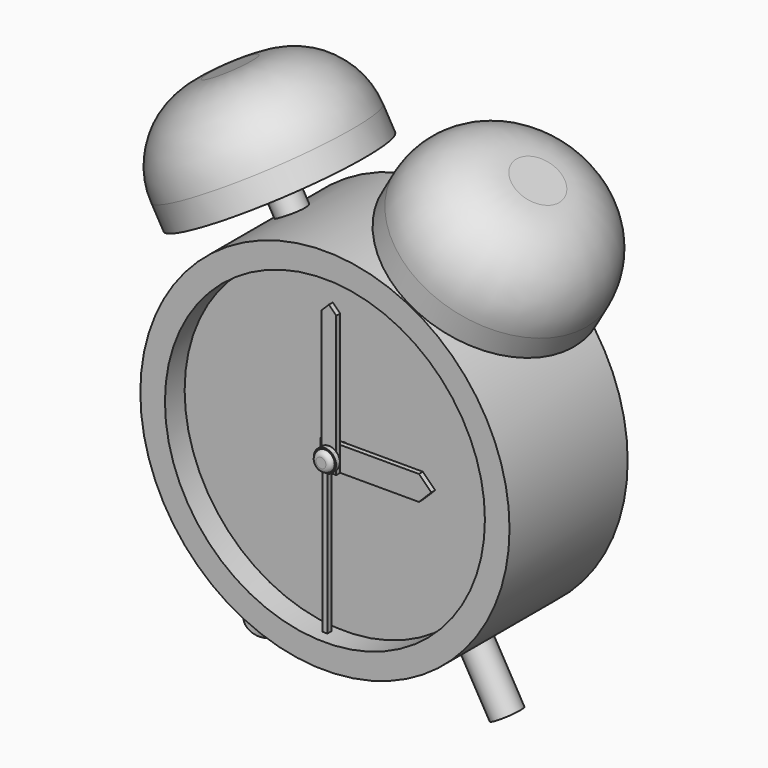
from build123d import *

# Parameters (mm, degrees)
F0_R      = 75
F1_DEPTH  = 60
F2_R      = 65
F3_DEPTH  = 10
F6_R      = 30
F7_ANGLE  = -30
F11_R     = 2.5
F12_DEPTH = 4
F14_DEPTH = 2
F15_SIZE  = 4.99999
F16_W     = 6
F16_H     = 50
F17_DEPTH = 2
F18_SIZE  = 2.99999
F19_W     = 2
F19_H     = 56.5
F20_DEPTH = 2
F21_DEPTH = 6
F22_R     = 4
F22_R_2   = 2.5
F23_DEPTH = 2
F24_R     = 1.99999


# Not quite as in the source:
# - a fillet or chamfer is up to 0.001 mm smaller than in the source, because OpenCascade refuses the exact size


with BuildPart() as f1:
    # F0 (on Front) → F1 (new body)
    with BuildSketch(Plane.XZ):
        Circle(F0_R)
    extrude(amount=F1_DEPTH)

    # F2 (on face) → F3 (cut)
    with BuildSketch(Plane.XZ.offset(60)):
        Circle(F2_R)
    extrude(amount=-F3_DEPTH, mode=Mode.SUBTRACT)


with BuildPart() as f5:
    # F4 (on Front) → F5 (revolve)
    with BuildSketch(Plane.XZ):
        Polygon((40, 125), (0, 125), (0, -100), (6, -100), (6, 85), (40, 85), align=None)
    revolve(axis=Axis((0, 0, 12.5), (0, 0, -1)))

    # F6
    f6_edges = [f5.edges().sort_by_distance(p)[0] for p in [
        (-40, 0, 125),
    ]]
    fillet(f6_edges, radius=F6_R)


with BuildPart() as f5_1:
    # F7: moved
    add(f5.part.rotate(Axis((0, 0, 0), (0, -1, 0)), F7_ANGLE))


with BuildPart() as f5_2:
    # F8: moved
    add(f5_1.part.moved(Location((0, -30, 0))))


with BuildPart() as f9_1:
    # F9: instance of F5
    add(f5_2.part.mirror(Plane.YZ))


with BuildPart() as f1_1:
    add(f1.part)

    # F10: cut F5, F9_1
    add(f5_2.part, mode=Mode.SUBTRACT)
    add(f9_1.part, mode=Mode.SUBTRACT)

    # F11 (on face) → F12 (join)
    with BuildSketch(Plane.XZ.offset(50)):
        Circle(F11_R)
    extrude(amount=F12_DEPTH)


with BuildPart() as f14:
    # F13 (on face) → F14 (new body)
    with BuildSketch(Plane.XZ.offset(54)):
        Polygon((40, 5), (-5, 5), (-5, 0), (-5, -5), (40, -5), align=None)
        with BuildLine():
            ThreePointArc((2.5, 0), (0, -2.5), (-2.5, 0))
            ThreePointArc((-2.5, 0), (0, 2.5), (2.5, 0))
        make_face(mode=Mode.SUBTRACT)
    extrude(amount=F14_DEPTH)

    # F15 (size 5 in the source; OpenCascade refuses exactly that, so slightly less here)
    f15_edges = [f14.edges().sort_by_distance(p)[0] for p in [
        (40, -55, 5),
        (40, -55, -5),
    ]]
    chamfer(f15_edges, length=F15_SIZE)

    # F16 (on face) → F17 (join)
    with BuildSketch(Plane.XZ.offset(56)):
        with Locations((0, 30)):
            Rectangle(F16_W, F16_H)
        Polygon((-3, 5), (-3, -5), (0, -5), (3, -5), (3, 5), align=None)
        with BuildLine():
            ThreePointArc((2.5, 0), (1.767766953, -1.767766953), (0, -2.5))
            ThreePointArc((0, -2.5), (-1.767766953, 1.767766953), (2.5, 0))
        make_face(mode=Mode.SUBTRACT)
    extrude(amount=F17_DEPTH)

    # F18 (size 3 in the source; OpenCascade refuses exactly that, so slightly less here)
    f18_edges = [f14.edges().sort_by_distance(p)[0] for p in [
        (3, -57, 55),
        (-3, -57, 55),
    ]]
    chamfer(f18_edges, length=F18_SIZE)


with BuildPart() as f20:
    # F19 (on face) → F20 (new body)
    with BuildSketch(Plane.XZ.offset(58)):
        with BuildLine():
            Line((3, -3.3541019662), (3, 3.3541019662))
            ThreePointArc((3, 3.3541019662), (0, 4.5), (-3, 3.3541019662))
            Line((-3, 3.3541019662), (-3, -3.3541019662))
            ThreePointArc((-3, -3.3541019662), (-2.0656642209, -3.9978783531), (-1, -4.3874821937))
            Line((-1, -4.3874821937), (-1, -2.2912878475))
            ThreePointArc((-1, -2.2912878475), (-1.3693063938, 2.0916500663), (2.5, 0))
            ThreePointArc((2.5, 0), (2.0916500663, -1.3693063938), (1, -2.2912878475))
            Line((1, -2.2912878475), (1, -4.3874821937))
            ThreePointArc((1, -4.3874821937), (2.0656642209, -3.9978783531), (3, -3.3541019662))
        make_face()
        with BuildLine():
            ThreePointArc((3, -3.3541019662), (4.1079191813, -1.8371173071), (4.5, 0))
            ThreePointArc((4.5, 0), (4.1079191813, 1.8371173071), (3, 3.3541019662))
            Line((3, 3.3541019662), (3, -3.3541019662))
        make_face()
        with BuildLine():
            Line((-3, -3.3541019662), (-3, 3.3541019662))
            ThreePointArc((-3, 3.3541019662), (-4.5, 0), (-3, -3.3541019662))
        make_face()
        with BuildLine():
            ThreePointArc((-1, -4.3874821937), (0, -4.5), (1, -4.3874821937))
            Line((1, -4.3874821937), (1, -2.2912878475))
            ThreePointArc((1, -2.2912878475), (0, -2.5), (-1, -2.2912878475))
            Line((-1, -2.2912878475), (-1, -4.3874821937))
        make_face()
        with Locations((0, -33.25)):
            Rectangle(F19_W, F19_H)
        with BuildLine():
            Line((1, -5), (1, -4.3874821937))
            ThreePointArc((1, -4.3874821937), (0, -4.5), (-1, -4.3874821937))
            Line((-1, -4.3874821937), (-1, -5))
            Line((-1, -5), (1, -5))
        make_face()
    extrude(amount=F20_DEPTH)


with BuildPart() as f21:
    # F21 (new, through all): a face of the model
    f21_faces = [f1_1.part.faces().sort_by_distance(p)[0] for p in [
        (0, -54, 0),
    ]]
    extrude(f21_faces, amount=F21_DEPTH)

    # F22 (on face) → F23 (join)
    with BuildSketch(Plane.XZ.offset(60)):
        Circle(F22_R)
        Circle(F22_R_2, mode=Mode.SUBTRACT)
        Circle(F22_R_2)
    extrude(amount=F23_DEPTH)

    # F24 (radius 2 in the source; OpenCascade refuses exactly that, so slightly less here)
    f24_edges = [f21.edges().sort_by_distance(p)[0] for p in [
        (-4, -62, 0),
    ]]
    fillet(f24_edges, radius=F24_R)


solid = Compound([f5_2.part, f9_1.part, f1_1.part, f14.part, f20.part, f21.part])
